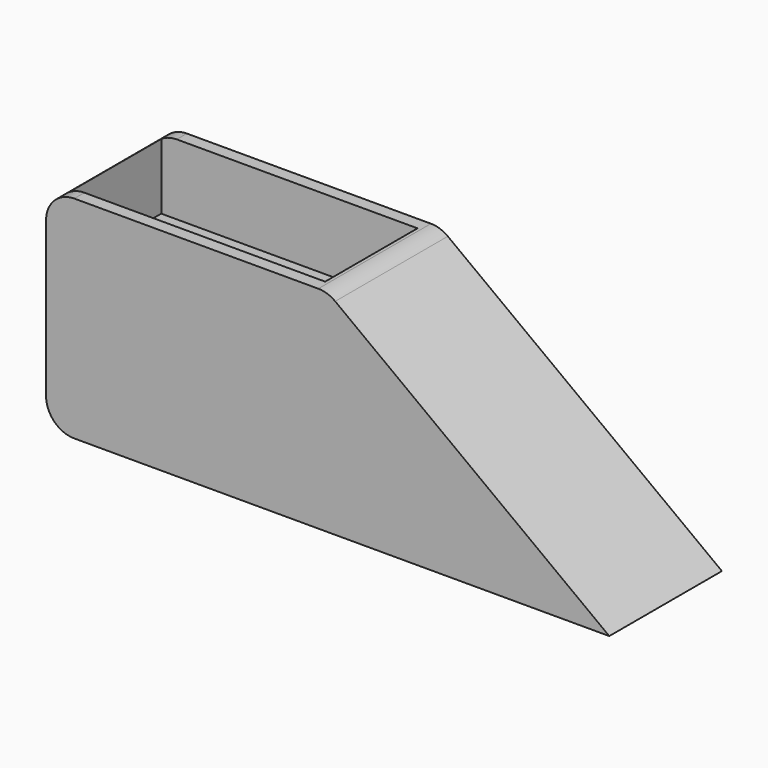
from build123d import *

# Parameters (mm, degrees)
F1_DEPTH    = 25.4
F2_W        = 46.228
F2_H        = 20.828
F3_DEPTH    = 12.7
F4_T1_DEPTH = 50.8
F4_T3_DEPTH = 33.8666666667


# Not quite as in the source:
# - a fillet or chamfer that OpenCascade refuses, or shapes differently, is made with other operations: its cross-section is extruded or revolved along the edge and cut away or added


with BuildPart() as f1:
    # F0 (on Front) → F1 (new body)
    with BuildSketch(Plane.XZ):
        Polygon((0, 38.1), (0, 0), (101.6, 0), (50.8, 38.1), align=None)
    extrude(amount=F1_DEPTH)

    # F2 (on face) → F3 (cut)
    with BuildSketch(Plane.XY.offset(38.1)):
        with Locations((25.4, -12.7)):
            Rectangle(F2_W, F2_H)
    extrude(amount=-F3_DEPTH, mode=Mode.SUBTRACT)

    # F4: fillet of radius 5.08 on 3 edges, made by hand

    # F4_s2 → F4_t1 (cut)
    with BuildSketch(Plane.XZ.offset(-12.7)):
        with BuildLine():
            ThreePointArc((0, 33.02), (1.4878975516, 36.6121024484), (5.08, 38.1))
            Line((5.08, 38.1), (0, 38.1))
            Line((0, 38.1), (0, 33.02))
        make_face()
        with BuildLine():
            ThreePointArc((0, 5.08), (1.4878975516, 1.4878975516), (5.08, 0))
            Line((5.08, 0), (0, 0))
            Line((0, 0), (0, 5.08))
        make_face()
    extrude(amount=F4_T1_DEPTH, mode=Mode.SUBTRACT)

    # F4_s4 → F4_t3 (cut)
    with BuildSketch(Plane.XZ.offset(-4.2333333333)):
        with BuildLine():
            ThreePointArc((49.1066666667, 38.1), (50.713103718, 37.8393111541), (52.1546666667, 37.084))
            Line((52.1546666667, 37.084), (50.8, 38.1))
            Line((50.8, 38.1), (49.1066666667, 38.1))
        make_face()
    extrude(amount=F4_T3_DEPTH, mode=Mode.SUBTRACT)


solid = f1.part
